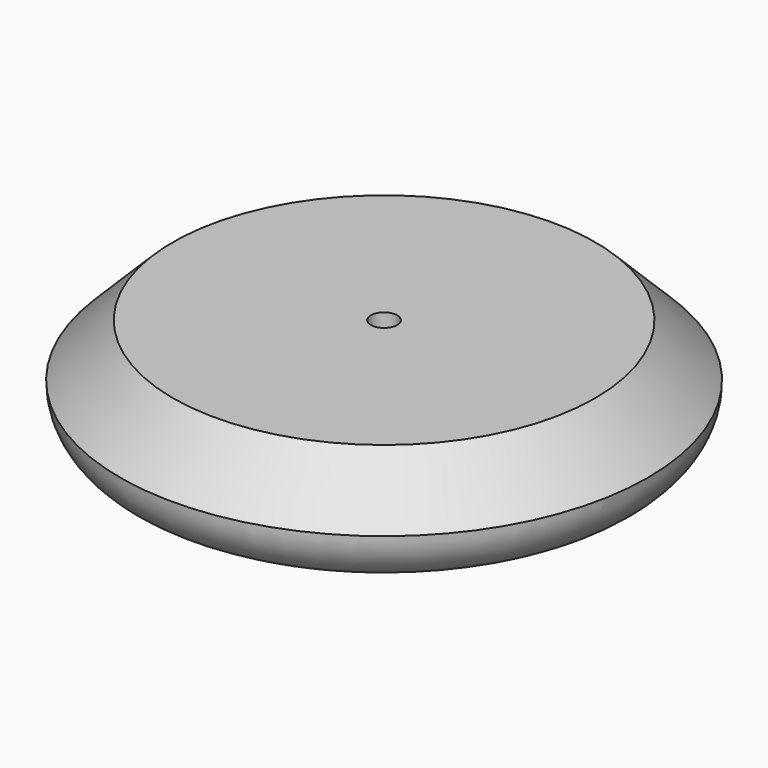
from build123d import *

# Parameters (mm, degrees)
F0_R     = 25.4
F1_DEPTH = 10.16
F2_R     = 1.27
F3_DEPTH = 5.08
F4_SIZE  = 5.08
F5_R     = 5.07999
F6_T     = 2.54


# Not quite as in the source:
# - a fillet or chamfer is up to 0.001 mm smaller than in the source, because OpenCascade refuses the exact size
# - a shell that OpenCascade refuses in one call is made with other operations: the cavity is built on its own and cut out


with BuildPart() as f1:
    # F0 (on Top) → F1 (new body)
    with BuildSketch(Plane.XY):
        Circle(F0_R)
    extrude(amount=F1_DEPTH)

    # F2 (on face) → F3 (cut)
    with BuildSketch(Plane.XY.offset(10.16)):
        Circle(F2_R)
    extrude(amount=-F3_DEPTH, mode=Mode.SUBTRACT)

    # F4
    f4_edges = [f1.edges().sort_by_distance(p)[0] for p in [
        (-25.4, 0, 10.16),
    ]]
    chamfer(f4_edges, length=F4_SIZE)

    # F5 (radius 5.08 in the source; OpenCascade refuses exactly that, so slightly less here)
    f5_edges = [f1.edges().sort_by_distance(p)[0] for p in [
        (-25.4, 0, 0),
    ]]
    fillet(f5_edges, radius=F5_R)

    # F6: shell of thickness 2.54, made by hand


with BuildPart() as f6_core1:
    # F6_t2: copy of F1
    add(f1.part)

    # the walls: a layer under each face that stays
    f6_faces = [f6_core1.faces().sort_by_distance(p)[0] for p in [
        (-25.4, 0, 5.079995),
        (-23.9121053774, 0, 1.4878946226),
        (-22.86, 0, 7.62),
        (-13.5466666667, -13.5466666667, 10.16),
        (-1.27, 0, 7.62),
        (0, 0, 5.08),
    ]]
    thicken(f6_faces, amount=-F6_T, mode=Mode.SUBTRACT)

    # F6_s3 → F6_t4 (revolve, cut)
    with BuildSketch(Plane.XZ):
        Polygon((1.2446, 5.1054), (3.81, 5.08), (3.81, 2.54), (1.27, 2.54), align=None)
    revolve(axis=Axis((0, 0, 5.08), (0, 0, 1)), mode=Mode.SUBTRACT)


with BuildPart() as f1_1:
    add(f1.part)

    # what is left inside the walls is the cavity
    f6_cavity = [f6_core1.part.solids().sort_by_distance(p)[0] for p in [
        (0, -6.773337, 0.0254),
    ]]
    add(f6_cavity, mode=Mode.SUBTRACT)


solid = f1_1.part
